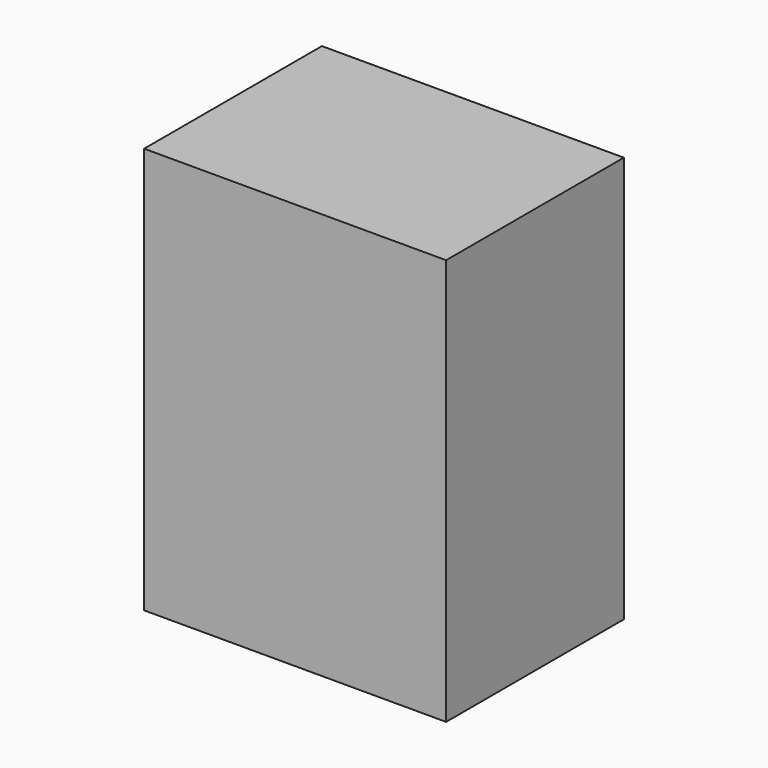
from build123d import *

# Parameters (mm, degrees)
F0_W     = 34.5230773091
F0_H     = 46.4703068137
F1_DEPTH = 25.4


# Not quite as in the source:
# - a feature names something its author has since deleted; it is built from what else it names


with BuildPart() as f1:
    # F0 (on Front) → F1 (new body)
    with BuildSketch(Plane.XZ):
        with Locations((-17.2615386546, 23.2351534069)):
            Rectangle(F0_W, F0_H)
    extrude(amount=F1_DEPTH)


solid = f1.part
